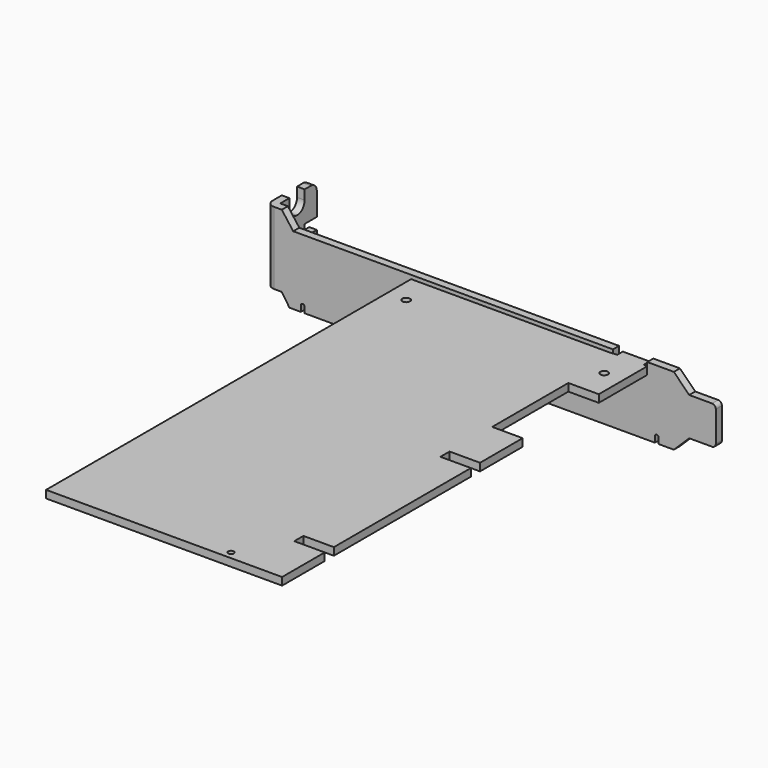
from build123d import *

# Parameters (mm, degrees)
F0_W      = 8
F0_H      = 16
F0_H_2    = 14
F0_H_3    = 45
F1_DEPTH  = 2
F2_W      = 20
F2_H      = 15
F3_DEPTH  = 3
F5_DEPTH  = 4
F6_R      = 0.75
F7_DEPTH  = 25
F8_R      = 1
F9_DEPTH  = 25
F11_DEPTH = 9
F12_SIZE  = 3.5
F13_SIZE  = 3.5
F14_R     = 1
F15_R     = 1
F17_W     = 7
F17_H     = 1.5
F18_DEPTH = 14
F19_DEPTH = 2
F20_W     = 7
F20_H     = 1.5
F21_DEPTH = 14
F22_DEPTH = 2
F24_DEPTH = 9
F26_DEPTH = 9
F29_DEPTH = 2
F31_DEPTH = 12
F32_R     = 2
F33_R     = 2
F34_W     = 4
F34_H     = 3
F35_DEPTH = 25
F37_DEPTH = 25


# Not quite as in the source:
# - two fillets or chamfers of one size are made in one step


with BuildPart() as f1:
    # F0 (on Top) → F1 (new body)
    with BuildSketch(Plane.XY):
        Polygon((22.8202738762, 74.1253000498), (-31.1797261238, 74.1253000498), (-31.1797261238, -45.8746999502), (22.8202738762, -45.8746999502), (22.8202738762, -31.8746999502), (22.8202738762, -28.8746999502), (22.8202738762, 16.1253000498), (22.8202738762, 19.1253000498), (22.8202738762, 33.1253000498), (22.8202738762, 58.1253000498), align=None)
        with Locations((26.8202738762, 66.1253000498)):
            Rectangle(F0_W, F0_H)
        with Locations((26.8202738762, -38.8746999502)):
            Rectangle(F0_W, F0_H_2)
        with Locations((26.8202738762, 26.1253000498)):
            Rectangle(F0_W, F0_H_2)
        with Locations((26.8202738762, -6.3746999502)):
            Rectangle(F0_W, F0_H_3)
    extrude(amount=F1_DEPTH)

    # F2 (on face) → F3 (join)
    with BuildSketch(Plane.XY.offset(2)):
        with Locations((5.8202738762, -6.3746999502)):
            Rectangle(F2_W, F2_H)
    extrude(amount=-F3_DEPTH)

    # F4 (on face) → F5 (join)
    with BuildSketch(Plane(origin=(0, 0, 0), x_dir=(1, 0, 0), z_dir=(0, 0, -1))):
        with BuildLine():
            ThreePointArc((-4.1797261238, -13.6253000498), (-4.619065952, -12.564639878), (-5.6797261238, -12.1253000498))
            Line((-5.6797261238, -12.1253000498), (-12.6797261238, -12.1253000498))
            ThreePointArc((-12.6797261238, -12.1253000498), (-13.7403862956, -12.564639878), (-14.1797261238, -13.6253000498))
            ThreePointArc((-14.1797261238, -13.6253000498), (-13.7403862956, -14.6859602216), (-12.6797261238, -15.1253000498))
            Line((-12.6797261238, -15.1253000498), (-5.6797261238, -15.1253000498))
            ThreePointArc((-5.6797261238, -15.1253000498), (-4.619065952, -14.6859602216), (-4.1797261238, -13.6253000498))
        make_face()
    extrude(amount=F5_DEPTH)

    # F6 (on face) → F7 (cut)
    with BuildSketch(Plane(origin=(0, 0, 0), x_dir=(1, 0, 0), z_dir=(0, 0, -1))):
        with Locations((15.8202738762, 43.8746999502)):
            Circle(F6_R)
    extrude(amount=-F7_DEPTH, mode=Mode.SUBTRACT)

    # F8 (on face) → F9 (cut)
    with BuildSketch(Plane(origin=(0, 0, 0), x_dir=(1, 0, 0), z_dir=(0, 0, -1))):
        with Locations((25.8202738762, -66.1253000498)):
            Circle(F8_R)
        with Locations((-26.1797261238, -66.1253000498)):
            Circle(F8_R)
    extrude(amount=-F9_DEPTH, mode=Mode.SUBTRACT)

    # F10 (on face) → F11 (join)
    with BuildSketch(Plane(origin=(0, 0, 0), x_dir=(1, 0, 0), z_dir=(0, 0, -1))):
        Polygon((14.8202738762, -76.1253000498), (14.8202738762, -74.1253000498), (14.8202738762, -61.1253000498), (1.8202738762, -61.1253000498), (1.8202738762, -74.1253000498), (1.8202738762, -76.1253000498), align=None)
        Polygon((-15.1797261238, -61.1253000498), (-15.1797261238, -74.1253000498), (-15.1797261238, -76.1253000498), (-2.1797261238, -76.1253000498), (-2.1797261238, -74.1253000498), (-2.1797261238, -61.1253000498), align=None)
    extrude(amount=F11_DEPTH)

    # F12
    f12_edges = [f1.edges().sort_by_distance(p)[0] for p in [
        (14.820274, 68.6253, -9),
    ]]
    chamfer(f12_edges, length=F12_SIZE)

    # F13
    f13_edges = [f1.edges().sort_by_distance(p)[0] for p in [
        (14.820274, 75.1253, 0),
        (-2.179726, 75.1253, 0),
        (-2.179726, 68.6253, -9),
    ]]
    chamfer(f13_edges, length=F13_SIZE)

    # F14
    f14_edges = [f1.edges().sort_by_distance(p)[0] for p in [
        (1.820274, 68.6253, -9),
    ]]
    fillet(f14_edges, radius=F14_R)

    # F15
    f15_edges = [f1.edges().sort_by_distance(p)[0] for p in [
        (-15.179726, 68.6253, -9),
    ]]
    fillet(f15_edges, radius=F15_R)

    # F17 (on face) → F18 (cut)
    with BuildSketch(Plane(origin=(0, 76.1253000498, 0), x_dir=(-1, 0, 0), z_dir=(0, 1, 0))):
        Polygon((14.1797261238, -8), (14.1797261238, -1), (5.6797261238, -1), (3.1797261238, -3.5), (3.1797261238, -5.5), (5.6797261238, -8), align=None)
        with Locations((9.1797261238, -4.75)):
            Rectangle(F17_W, F17_H, mode=Mode.SUBTRACT)
    extrude(amount=-F18_DEPTH, mode=Mode.SUBTRACT)

    # F19 (cut): a face of the model
    f19_faces = [f1.faces().sort_by_distance(p)[0] for p in [
        (-9.1797261238, 76.1253000498, -4.75),
    ]]
    extrude(f19_faces, amount=-F19_DEPTH, mode=Mode.SUBTRACT)

    # F20 (on face) → F21 (cut)
    with BuildSketch(Plane(origin=(0, 76.1253000498, 0), x_dir=(-1, 0, 0), z_dir=(0, 1, 0))):
        Polygon((-2.8202738762, -8), (-2.8202738762, -4), (-2.8202738762, -1), (-11.3202738762, -1), (-13.8202738762, -3.5), (-13.8202738762, -5.5), (-11.3202738762, -8), align=None)
        with Locations((-7.8202738762, -4.75)):
            Rectangle(F20_W, F20_H, mode=Mode.SUBTRACT)
    extrude(amount=-F21_DEPTH, mode=Mode.SUBTRACT)

    # F22 (cut): a face of the model
    f22_faces = [f1.faces().sort_by_distance(p)[0] for p in [
        (7.8202738762, 76.1253000498, -4.75),
    ]]
    extrude(f22_faces, amount=-F22_DEPTH, mode=Mode.SUBTRACT)

    # F23 (on face) → F24 (cut)
    with BuildSketch(Plane(origin=(0, 74.1253000498, 0), x_dir=(-1, 0, 0), z_dir=(0, 1, 0))):
        Polygon((-11.3202738762, 0), (-14.8202738762, 0), (-14.8202738762, -3.5), align=None)
    extrude(amount=-F24_DEPTH, mode=Mode.SUBTRACT)

    # F25 (on face) → F26 (cut)
    with BuildSketch(Plane(origin=(0, 74.1253000498, 0), x_dir=(-1, 0, 0), z_dir=(0, 1, 0))):
        Polygon((2.1797261238, -3.5), (5.6797261238, 0), (2.1797261238, 0), align=None)
    extrude(amount=-F26_DEPTH, mode=Mode.SUBTRACT)

    # F28 (on offset) → F29 (join)
    with BuildSketch(Plane.XZ.offset(-76)):
        with BuildLine():
            Line((21.8447855255, 3), (1.8447855255, 3))
            Line((1.8447855255, 3), (0, 3))
            Line((0, 3), (-62.1552144745, 3))
            Line((-62.1552144745, 3), (-65.1552144745, 7))
            Line((-65.1552144745, 7), (-69.1552144745, 7))
            Line((-69.1552144745, 7), (-69.1552144745, -4.8977956176))
            Line((-69.1552144745, -4.8977956176), (-69.1552144745, -12))
            Line((-69.1552144745, -12), (-65.1552144745, -12))
            Line((-65.1552144745, -12), (-63.1552144745, -15))
            Line((-63.1552144745, -15), (-60.1552144745, -15))
            Line((-60.1552144745, -15), (-60.1552144745, -13.5))
            ThreePointArc((-60.1552144745, -13.5), (-60.0087678651, -13.1464466094), (-59.6552144745, -13))
            ThreePointArc((-59.6552144745, -13), (-59.3016610839, -13.1464466094), (-59.1552144745, -13.5))
            Line((-59.1552144745, -13.5), (-59.1552144745, -15))
            Line((-59.1552144745, -15), (32.8447855255, -15))
            Line((32.8447855255, -15), (32.8447855255, -13.5))
            ThreePointArc((32.8447855255, -13.5), (32.9912321349, -13.1464466094), (33.3447855255, -13))
            ThreePointArc((33.3447855255, -13), (33.6983389161, -13.1464466094), (33.8447855255, -13.5))
            Line((33.8447855255, -13.5), (33.8447855255, -15))
            Line((33.8447855255, -15), (37.8447855255, -15))
            Line((37.8447855255, -15), (41.8670170307, -11.0439766385))
            Line((41.8670170307, -11.0439766385), (47.8670170307, -11.0439766385))
            ThreePointArc((47.8670170307, -11.0439766385), (48.5741238119, -10.7510834197), (48.8670170307, -10.0439766385))
            Line((48.8670170307, -10.0439766385), (48.8670170307, -6.0439766385))
            Line((48.8670170307, -6.0439766385), (48.8670170307, -2.0439766385))
            ThreePointArc((48.8670170307, -2.0439766385), (48.5741238119, -1.3368698573), (47.8670170307, -1.0439766385))
            Line((47.8670170307, -1.0439766385), (41.8670170307, -1.0439766385))
            Line((41.8670170307, -1.0439766385), (37.8447855255, 3))
            Line((37.8447855255, 3), (30.8447855255, 3))
            Line((30.8447855255, 3), (30.8447855255, 0.5))
            ThreePointArc((30.8447855255, 0.5), (30.6983389161, 0.1464466094), (30.3447855255, 0))
            ThreePointArc((30.3447855255, 0), (29.9912321349, 0.1464466094), (29.8447855255, 0.5))
            Line((29.8447855255, 0.5), (29.8447855255, 2))
            Line((29.8447855255, 2), (22.8447855255, 2))
            Line((22.8447855255, 2), (22.8447855255, 0.5))
            ThreePointArc((22.8447855255, 0.5), (22.6983389161, 0.1464466094), (22.3447855255, 0))
            ThreePointArc((22.3447855255, 0), (21.9912321349, 0.1464466094), (21.8447855255, 0.5))
            Line((21.8447855255, 0.5), (21.8447855255, 3))
        make_face()
        with BuildLine():
            Line((-5.1067974085, -9.6197371359), (-9.916828014, -9.6487514675))
            Line((-9.916828014, -9.6487514675), (-14.5359628499, -9.6487514675))
            ThreePointArc((-14.5359628499, -9.6487514675), (-15.5966230216, -9.2094116392), (-16.0359628499, -8.1487514675))
            Line((-16.0359628499, -8.1487514675), (-16.0359628499, -4.194740206))
            Line((-16.0359628499, -4.194740206), (-16.0359628499, -0.8))
            ThreePointArc((-16.0359628499, -0.8), (-15.5966230216, 0.2606601718), (-14.5359628499, 0.7))
            Line((-14.5359628499, 0.7), (-9.4512412325, 0.7))
            Line((-9.4512412325, 0.7), (-5.5935280398, 0.7))
            Line((-5.5935280398, 0.7), (-1.5013976704, -3.5296175629))
            Line((-1.5013976704, -3.5296175629), (-1.5013976704, -5.5249878205))
            Line((-1.5013976704, -5.5249878205), (-5.1067974085, -9.6197371359))
        make_face(mode=Mode.SUBTRACT)
        with BuildLine():
            Line((15.5488683626, -5.5253235623), (11.2658282742, -9.6197371359))
            Line((11.2658282742, -9.6197371359), (2.5931737488, -9.6197371359))
            ThreePointArc((2.5931737488, -9.6197371359), (1.532513577, -9.1803973077), (1.0931737488, -8.1197371359))
            Line((1.0931737488, -8.1197371359), (1.0931737488, -4.0044868365))
            Line((1.0931737488, -4.0044868365), (1.0931737488, -0.8))
            ThreePointArc((1.0931737488, -0.8), (1.532513577, 0.2606601718), (2.5931737488, 0.7))
            Line((2.5931737488, 0.7), (7.3360428214, 0.7))
            Line((7.3360428214, 0.7), (11.4213749766, 0.7))
            Line((11.4213749766, 0.7), (15.5199731484, -3.473744262))
            Line((15.5199731484, -3.473744262), (15.5488683626, -5.5253235623))
        make_face(mode=Mode.SUBTRACT)
    extrude(amount=F29_DEPTH)

    # F30 (on face) → F31 (join)
    with BuildSketch(Plane(origin=(0, 76, 0), x_dir=(-1, 0, 0), z_dir=(0, 1, 0))):
        Polygon((67.1552144745, 7), (67.1552144745, -5.6737242267), (67.1552144745, -12), (69.1552144745, -12), (69.1552144745, 7), align=None)
    extrude(amount=F31_DEPTH)

    # F32
    f32_edges = [f1.edges().sort_by_distance(p)[0] for p in [
        (-68.155214, 88, -12),
        (-68.155214, 88, 7),
    ]]
    fillet(f32_edges, radius=F32_R)

    # F33
    f33_edges = [f1.edges().sort_by_distance(p)[0] for p in [
        (-69.155214, 74, -2.5),
    ]]
    fillet(f33_edges, radius=F33_R)

    # F34 (on face) → F35 (cut)
    with BuildSketch(Plane(origin=(-69.1552144745, 0, 0), x_dir=(0, -1, 0), z_dir=(-1, 0, 0))):
        with Locations((-86, -2.5)):
            Rectangle(F34_W, F34_H)
    extrude(amount=-F35_DEPTH, mode=Mode.SUBTRACT)

    # F36 (on face) → F37 (cut)
    with BuildSketch(Plane(origin=(-69.1552144745, 0, 0), x_dir=(0, -1, 0), z_dir=(-1, 0, 0))):
        with BuildLine():
            Line((-79, 7), (-84, 7))
            Line((-84, 7), (-84, 4.5))
            ThreePointArc((-84, 4.5), (-83.267766953, 2.732233047), (-81.5, 2))
            ThreePointArc((-81.5, 2), (-79.732233047, 2.732233047), (-79, 4.5))
            Line((-79, 4.5), (-79, 7))
        make_face()
    extrude(amount=-F37_DEPTH, mode=Mode.SUBTRACT)


solid = f1.part
